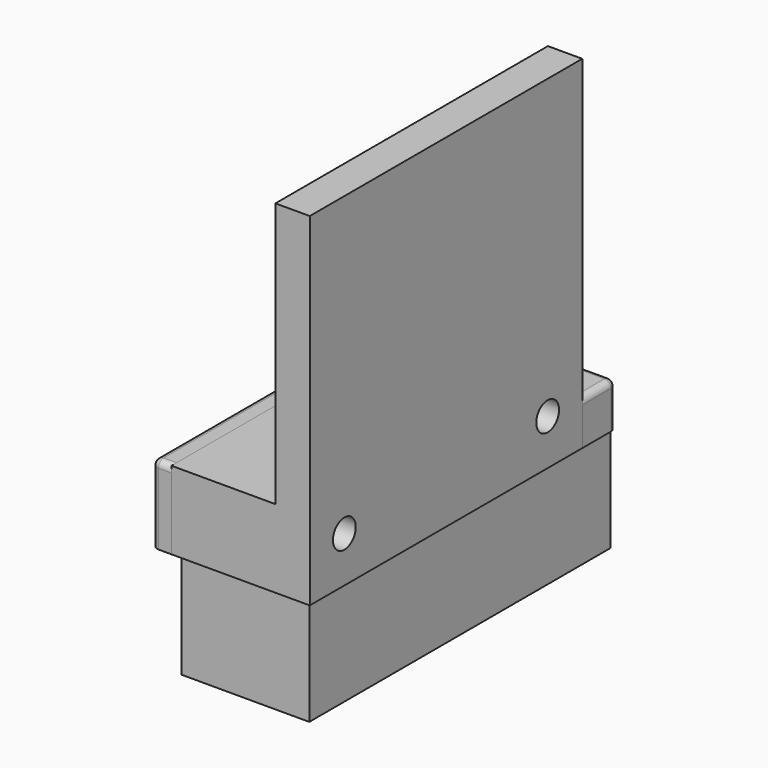
from build123d import *

# Parameters (mm, degrees)
F0_W      = 17.11
F0_H      = 42.13
F1_DEPTH  = 9.65
F3_W      = 42.13
F3_H      = 42.4
F4_DEPTH  = 4.25
F2_R      = 1.76
F5_DEPTH  = 17.111
F6_R      = 3
F7_DEPTH  = 25
F8_W      = 15.8
F8_H      = 46.6
F9_DEPTH  = 13.2
F10_R     = 3
F10_R_2   = 1.5
F11_DEPTH = 25
F12_W     = 42.13
F12_H     = 9.65
F12_R     = 1.76
F12_W_2   = 5.2117788947
F12_W_3   = 47.3417788947
F13_DEPTH = 2.4
F14_W     = 5.1398039788
F14_H     = 9.65
F15_DEPTH = 17.11
F16_R     = 1.5
F17_DEPTH = 25
F18_W     = 17.11
F18_H     = 5.1398039788
F19_DEPTH = 4.15
F20_R     = 0.8


with BuildPart() as f1:
    # F0 (on Top) → F1 (new body)
    with BuildSketch(Plane.XY):
        Rectangle(F0_W, F0_H)
    extrude(amount=F1_DEPTH)

    # F3 (on face) → F4 (join)
    with BuildSketch(Plane.YZ.offset(8.555)):
        with Locations((0, 21.2)):
            Rectangle(F3_W, F3_H)
    extrude(amount=-F4_DEPTH)

    # F2 (on face) → F5 (cut, through all)
    with BuildSketch(Plane(origin=(-8.555, 0, 0), x_dir=(0, -1, 0), z_dir=(-1, 0, 0))):
        with Locations((-15.715, 5.65)):
            Circle(F2_R)
        with Locations((15.715, 5.65)):
            Circle(F2_R)
    extrude(amount=-F5_DEPTH, mode=Mode.SUBTRACT)

    # F6 (on face) → F7 (cut)
    with BuildSketch(Plane(origin=(0, 0, 0), x_dir=(1, 0, 0), z_dir=(0, 0, -1))):
        with Locations((-2.405, -6.065)):
            Circle(F6_R)
    extrude(amount=-F7_DEPTH, mode=Mode.SUBTRACT)


with BuildPart() as f9:
    # F8 (on Top) → F9 (new body)
    with BuildSketch(Plane.XY):
        with Locations((0, 2.9767788947)):
            Rectangle(F8_W, F8_H)
    extrude(amount=-F9_DEPTH)

    # F10 (on face) → F11 (cut)
    with BuildSketch(Plane(origin=(0, 0, -13.2), x_dir=(1, 0, 0), z_dir=(0, 0, -1))):
        with Locations((-1.65, -5.9267788947)):
            Circle(F10_R)
        with Locations((-4.9, -23.2767788947)):
            Circle(F10_R_2)
        with Locations((4.9, -23.2767788947)):
            Circle(F10_R_2)
    extrude(amount=-F11_DEPTH, mode=Mode.SUBTRACT)


with BuildPart() as f13:
    # F12 (on face) → F13 (new body)
    with BuildSketch(Plane(origin=(-8.555, 0, 0), x_dir=(0, -1, 0), z_dir=(-1, 0, 0))):
        with Locations((0, 4.825)):
            Rectangle(F12_W, F12_H)
        with Locations((-15.715, 5.65)):
            Circle(F12_R, mode=Mode.SUBTRACT)
        with Locations((15.715, 5.65)):
            Circle(F12_R, mode=Mode.SUBTRACT)
        with Locations((-23.6708894473, 4.825)):
            Rectangle(F12_W_2, F12_H)
        with Locations((-2.6058894473, 4.825)):
            Rectangle(F12_W_3, F12_H)
        with Locations((-15.715, 5.65)):
            Circle(F12_R, mode=Mode.SUBTRACT)
        with Locations((15.715, 5.65)):
            Circle(F12_R, mode=Mode.SUBTRACT)
    extrude(amount=F13_DEPTH)

    # F14 (on face) → F15 (join, through all)
    with BuildSketch(Plane.YZ.offset(-8.555)):
        with Locations((23.7068769053, 4.825)):
            Rectangle(F14_W, F14_H)
    extrude(amount=F15_DEPTH)

    # F16 (on face) → F17 (cut)
    with BuildSketch(Plane.XY.offset(9.65)):
        with Locations((-4.9, 23.2767788947)):
            Circle(F16_R)
        with Locations((4.9, 23.2767788947)):
            Circle(F16_R)
    extrude(amount=-F17_DEPTH, mode=Mode.SUBTRACT)

    # F18 (on face) → F19 (cut)
    with BuildSketch(Plane.XY.offset(9.65)):
        with Locations((0, 23.7068769053)):
            Rectangle(F18_W, F18_H)
    extrude(amount=-F19_DEPTH, mode=Mode.SUBTRACT)

    # F20
    f20_edges = [f13.edges().sort_by_distance(p)[0] for p in [
        (8.555, 23.706877, 5.5),
        (0, 26.276779, 5.5),
        (-8.555, 23.706877, 5.5),
        (-8.555, 26.276779, 7.575),
        (-9.755, 26.276779, 9.65),
        (-10.955, 2.605889, 9.65),
        (-10.955, -21.065, 4.825),
        (-9.755, -21.065, 9.65),
        (8.555, 26.276779, 2.75),
        (-10.955, 26.276779, 4.825),
    ]]
    fillet(f20_edges, radius=F20_R)


solid = Compound([f1.part, f9.part, f13.part])
